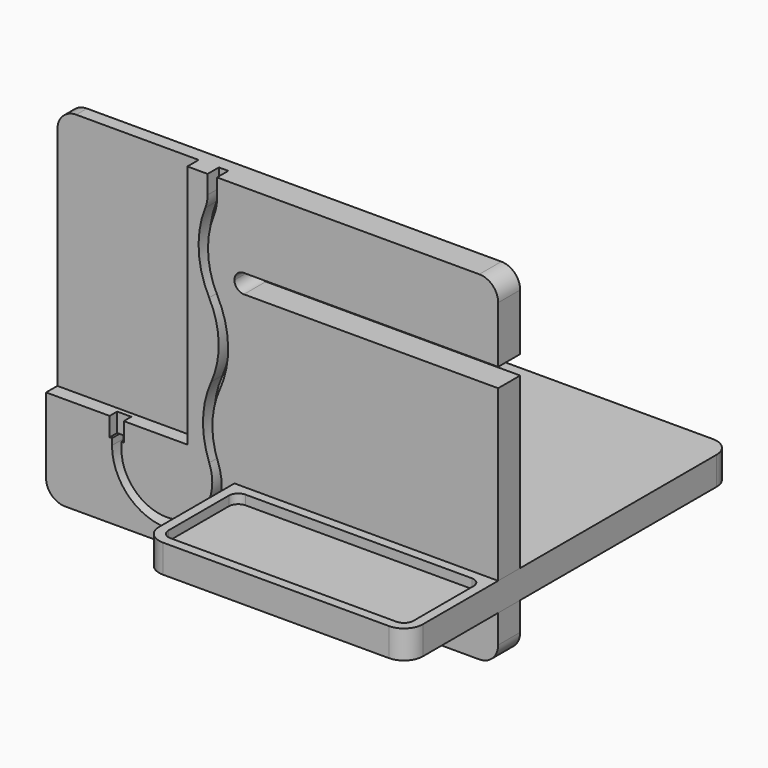
from build123d import *

# Parameters (mm, degrees)
F0_W           = 304.8
F0_H           = 228.6
F1_DEPTH       = 18.542
F2_W           = 177.8
F2_H           = 12.7
F2_W_2         = 76.2
F2_H_2         = 19.05
F3_DEPTH       = 18.543
F4_W           = 95.25
F4_H           = 165.1
F5_DEPTH       = 9.525
F6_W           = 9.525
F6_H           = 12.7
F7_DEPTH       = 6.35
F9_DEPTH       = 9.525
F10_R          = 12.7
F11_R          = 6.34999
F12_W          = 273.05
F12_H          = 19.05
F13_DEPTH      = 152.4
F13_DEPTH_BACK = 25.4
F14_W          = 18.542
F14_H          = 19.05
F15_DEPTH      = 111.125
F16_R          = 12.7
F17_R          = 3.175
F18_W          = 165.1
F18_H          = 63.5
F19_DEPTH      = 6.35
F20_R          = 6.35


# Not quite as in the source:
# - a fillet or chamfer is up to 0.001 mm smaller than in the source, because OpenCascade refuses the exact size


with BuildPart() as f1:
    # F0 (on Front) → F1 (new body)
    with BuildSketch(Plane.XZ):
        Rectangle(F0_W, F0_H)
    extrude(amount=-F1_DEPTH)

    # F2 (on face) → F3 (cut, through all)
    with BuildSketch(Plane.XZ):
        with Locations((63.5, 57.15)):
            Rectangle(F2_W, F2_H)
        with Locations((114.3, -73.025)):
            Rectangle(F2_W_2, F2_H_2)
    extrude(amount=-F3_DEPTH, mode=Mode.SUBTRACT)

    # F4 (on face) → F5 (cut)
    with BuildSketch(Plane.XZ):
        with Locations((-104.775, 31.75)):
            Rectangle(F4_W, F4_H)
    extrude(amount=-F5_DEPTH, mode=Mode.SUBTRACT)

    # F6 (on face) → F7 (cut)
    with BuildSketch(Plane.XZ):
        with Locations((-104.775, -57.15)):
            Rectangle(F6_W, F6_H)
    extrude(amount=-F7_DEPTH, mode=Mode.SUBTRACT)

    # F8 (on face) → F9 (cut)
    with BuildSketch(Plane.XZ):
        with BuildLine():
            ThreePointArc((-39.1997749684, 91.2285561772), (-37.6718013693, 96.4369674893), (-37.1562764049, 101.8403447412))
            Line((-37.1562764049, 101.8403447412), (-37.1562764049, 114.3))
            Line((-37.1562764049, 114.3), (-43.5062764049, 114.3))
            Line((-43.5062764049, 114.3), (-43.5062764049, 101.8403447412))
            ThreePointArc((-43.5062764049, 101.8403447412), (-43.9072402661, 97.6377179897), (-45.0956641765, 93.5867314137))
            ThreePointArc((-45.0956641765, 93.5867314137), (-49.5107233258, 67.0703536947), (-42.4445124385, 41.1342842484))
            ThreePointArc((-42.4445124385, 41.1342842484), (-36.0430844049, 16.5774501543), (-41.0339246807, -8.3044286924))
            ThreePointArc((-41.0339246807, -8.3044286924), (-46.586082977, -32.4137993186), (-42.4044952455, -56.7982726117))
            ThreePointArc((-42.4044952455, -56.7982726117), (-65.3759429594, -97.9182199908), (-101.6, -67.8124867486))
            Line((-101.6, -67.8124867486), (-101.6, -63.5))
            Line((-101.6, -63.5), (-107.95, -63.5))
            Line((-107.95, -63.5), (-107.95, -67.8124867486))
            ThreePointArc((-107.95, -67.8124867486), (-64.2143658736, -104.1610750006), (-36.4794594428, -54.5143175474))
            ThreePointArc((-36.4794594428, -54.5143175474), (-40.2386175991, -32.5931962998), (-35.2473457461, -10.9193864805))
            ThreePointArc((-35.2473457461, -10.9193864805), (-29.6956675249, 16.7585549608), (-36.8164461183, 44.0749252491))
            ThreePointArc((-36.8164461183, 44.0749252491), (-43.1688189483, 67.3908983351), (-39.1997749684, 91.2285561772))
        make_face()
    extrude(amount=-F9_DEPTH, mode=Mode.SUBTRACT)

    # F10
    f10_edges = [f1.edges().sort_by_distance(p)[0] for p in [
        (152.4, 9.271, 114.3),
        (152.4, 9.271, -114.3),
        (-152.4, 14.0335, 114.3),
        (-152.4, 9.271, -114.3),
    ]]
    fillet(f10_edges, radius=F10_R)

    # F11 (radius 6.35 in the source; OpenCascade refuses exactly that, so slightly less here)
    f11_edges = [f1.edges().sort_by_distance(p)[0] for p in [
        (-25.4, 9.271, 63.5),
        (-25.4, 9.271, 50.8),
        (76.2, 9.271, -82.55),
        (76.2, 9.271, -63.5),
    ]]
    fillet(f11_edges, radius=F11_R)


with BuildPart() as f13:
    # F12 (on Right) → F13 (new body, two sides)
    with BuildSketch(Plane.YZ) as f13_sk:
        with Locations((60.325, -73.025)):
            Rectangle(F12_W, F12_H)
    extrude(amount=F13_DEPTH)
    extrude(f13_sk.sketch, amount=-F13_DEPTH_BACK)

    # F14 (on face) → F15 (cut)
    with BuildSketch(Plane(origin=(-25.4, 0, 0), x_dir=(0, -1, 0), z_dir=(-1, 0, 0))):
        with Locations((-9.271, -73.025)):
            Rectangle(F14_W, F14_H)
    extrude(amount=-F15_DEPTH, mode=Mode.SUBTRACT)

    # F16
    f16_edges = [f13.edges().sort_by_distance(p)[0] for p in [
        (-25.4, -76.2, -73.025),
        (152.4, -76.2, -73.025),
        (152.4, 196.85, -73.025),
        (-25.4, 196.85, -73.025),
    ]]
    fillet(f16_edges, radius=F16_R)

    # F17
    f17_edges = [f13.edges().sort_by_distance(p)[0] for p in [
        (85.725, 18.542, -73.025),
        (85.725, 0, -73.025),
    ]]
    fillet(f17_edges, radius=F17_R)

    # F18 (on face) → F19 (cut)
    with BuildSketch(Plane.XY.offset(-63.5)):
        with Locations((63.5, -38.1)):
            Rectangle(F18_W, F18_H)
    extrude(amount=-F19_DEPTH, mode=Mode.SUBTRACT)

    # F20
    f20_edges = [f13.edges().sort_by_distance(p)[0] for p in [
        (-19.05, -69.85, -66.675),
        (-19.05, -6.35, -66.675),
        (146.05, -6.35, -66.675),
        (146.05, -69.85, -66.675),
    ]]
    fillet(f20_edges, radius=F20_R)


solid = Compound([f1.part, f13.part])
